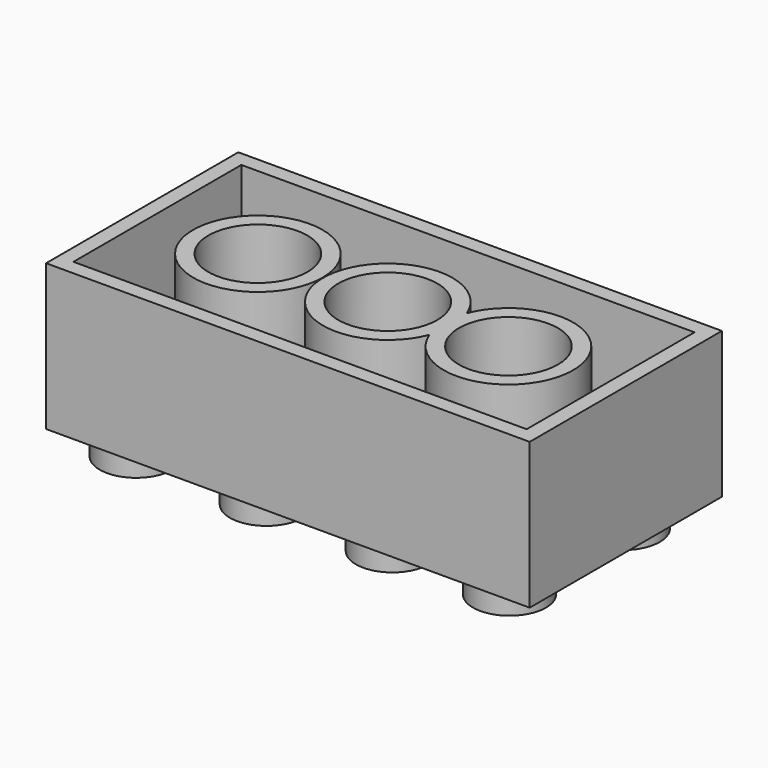
from build123d import *

# Parameters (mm, degrees)
F0_W     = 31.8
F0_H     = 15.8
F0_R     = 2.4
F0_R_2   = 3.255
F1_DEPTH = 9.6
F2_DEPTH = 1.6
F3_T     = -1


# Not quite as in the source:
# - a feature names something its author has since deleted; it is built from what else it names


with BuildPart() as f1:
    # F0 (on Top) → F1 (new body)
    with BuildSketch(Plane.XY):
        with Locations((-91.5395749569, 25.0114094891)):
            Rectangle(F0_W, F0_H)
        with Locations((-103.8533747765, 20.0384181401)):
            Circle(F0_R, mode=Mode.SUBTRACT)
        with Locations((-95.2911525131, 20.0384181401)):
            Circle(F0_R, mode=Mode.SUBTRACT)
        with Locations((-99.6062383056, 24.726472795)):
            Circle(F0_R_2, mode=Mode.SUBTRACT)
        with Locations((-87.0096325433, 20.0384181401)):
            Circle(F0_R, mode=Mode.SUBTRACT)
        with Locations((-79.3065652251, 20.0384181401)):
            Circle(F0_R, mode=Mode.SUBTRACT)
        with Locations((-91.0623019177, 24.726472795)):
            Circle(F0_R_2, mode=Mode.SUBTRACT)
        with Locations((-83.1293836236, 24.726472795)):
            Circle(F0_R_2, mode=Mode.SUBTRACT)
        with Locations((-103.5441160202, 29.3876323849)):
            Circle(F0_R, mode=Mode.SUBTRACT)
        with Locations((-95.5441160202, 29.3876323849)):
            Circle(F0_R, mode=Mode.SUBTRACT)
        with Locations((-87.0096325433, 29.3876323849)):
            Circle(F0_R, mode=Mode.SUBTRACT)
        with Locations((-79.3065652251, 29.3876323849)):
            Circle(F0_R, mode=Mode.SUBTRACT)
        with Locations((-103.5441160202, 29.3876323849)):
            Circle(F0_R)
        with Locations((-79.3065652251, 29.3876323849)):
            Circle(F0_R)
        with Locations((-87.0096325433, 29.3876323849)):
            Circle(F0_R)
        with Locations((-79.3065652251, 20.0384181401)):
            Circle(F0_R)
        with Locations((-103.8533747765, 20.0384181401)):
            Circle(F0_R)
        with Locations((-95.5441160202, 29.3876323849)):
            Circle(F0_R)
        with Locations((-95.2911525131, 20.0384181401)):
            Circle(F0_R)
        with Locations((-87.0096325433, 20.0384181401)):
            Circle(F0_R)
    extrude(amount=F1_DEPTH)

    # F3
    f3_openings = [f1.faces().sort_by_distance(p)[0] for p in [
        (-91.539575, 32.556321, 9.6),
    ]]
    offset(amount=F3_T, openings=f3_openings)


with BuildPart() as f2:
    # F0 (on Top) → F2 (new body)
    with BuildSketch(Plane.XY):
        with Locations((-103.5441160202, 29.3876323849)):
            Circle(F0_R)
    extrude(amount=-F2_DEPTH)


with BuildPart() as f2b:
    # F0 (on Top) → F2, piece 2 (new body)
    with BuildSketch(Plane.XY):
        with Locations((-87.0096325433, 29.3876323849)):
            Circle(F0_R)
    extrude(amount=-F2_DEPTH)


with BuildPart() as f2c:
    # F0 (on Top) → F2, piece 3 (new body)
    with BuildSketch(Plane.XY):
        with Locations((-95.5441160202, 29.3876323849)):
            Circle(F0_R)
    extrude(amount=-F2_DEPTH)


with BuildPart() as f2d:
    # F0 (on Top) → F2, piece 4 (new body)
    with BuildSketch(Plane.XY):
        with Locations((-79.3065652251, 29.3876323849)):
            Circle(F0_R)
    extrude(amount=-F2_DEPTH)


with BuildPart() as f2e:
    # F0 (on Top) → F2, piece 5 (new body)
    with BuildSketch(Plane.XY):
        with Locations((-87.0096325433, 20.0384181401)):
            Circle(F0_R)
    extrude(amount=-F2_DEPTH)


with BuildPart() as f2f:
    # F0 (on Top) → F2, piece 6 (new body)
    with BuildSketch(Plane.XY):
        with Locations((-79.3065652251, 20.0384181401)):
            Circle(F0_R)
    extrude(amount=-F2_DEPTH)


with BuildPart() as f2g:
    # F0 (on Top) → F2, piece 7 (new body)
    with BuildSketch(Plane.XY):
        with Locations((-95.2911525131, 20.0384181401)):
            Circle(F0_R)
    extrude(amount=-F2_DEPTH)


with BuildPart() as f2h:
    # F0 (on Top) → F2, piece 8 (new body)
    with BuildSketch(Plane.XY):
        with Locations((-103.8533747765, 20.0384181401)):
            Circle(F0_R)
    extrude(amount=-F2_DEPTH)


solid = Compound([f1.part, f2.part, f2b.part, f2c.part, f2d.part, f2e.part, f2f.part, f2g.part, f2h.part])
